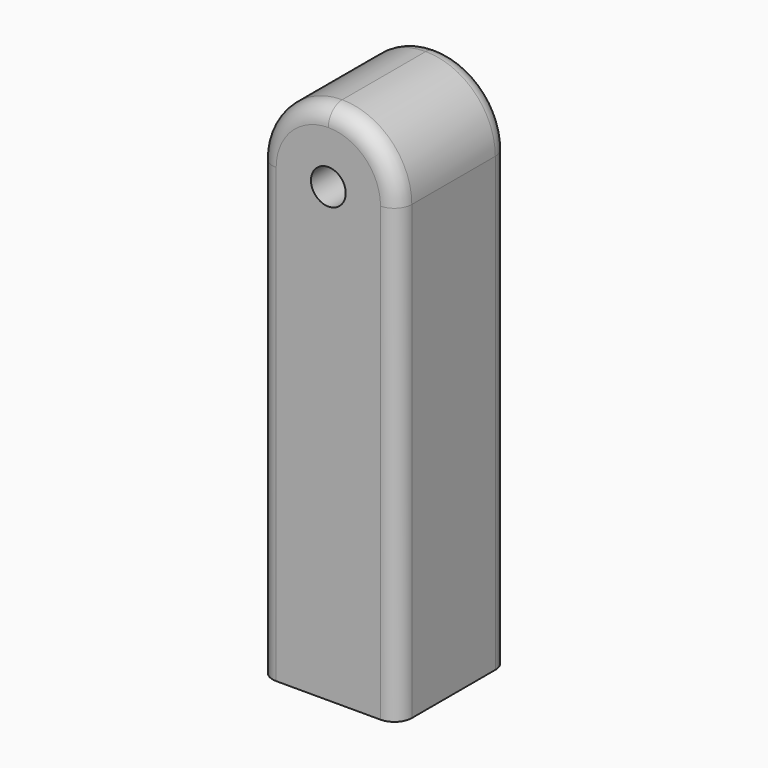
from build123d import *

# Parameters (mm, degrees)
F1_DEPTH = 40
F2_D     = 10
F3_R     = 5


with BuildPart() as f1:
    # F0 (on Front) → F1 (new body)
    with BuildSketch(Plane.XZ):
        with BuildLine():
            Line((-20, 55), (-20, -75))
            Line((-20, -75), (20, -75))
            Line((20, -75), (20, 55))
            ThreePointArc((20, 55), (14.1421356237, 69.1421356237), (0, 75))
            ThreePointArc((0, 75), (-14.1421356237, 69.1421356237), (-20, 55))
        make_face()
    extrude(amount=F1_DEPTH)

    # F2 (through all)
    with Locations(Plane(origin=(0, 0, 0), x_dir=(1, 0, 0), z_dir=(0, 1, 0))):
        with Locations((0, -55)):
            Hole(F2_D / 2)

    # F3
    f3_edges = [f1.edges().sort_by_distance(p)[0] for p in [
        (0, -40, 75),
        (0, 0, 75),
        (-20, 0, -10),
        (-20, -40, -10),
        (20, 0, -10),
        (20, -40, -10),
    ]]
    fillet(f3_edges, radius=F3_R)


solid = f1.part
